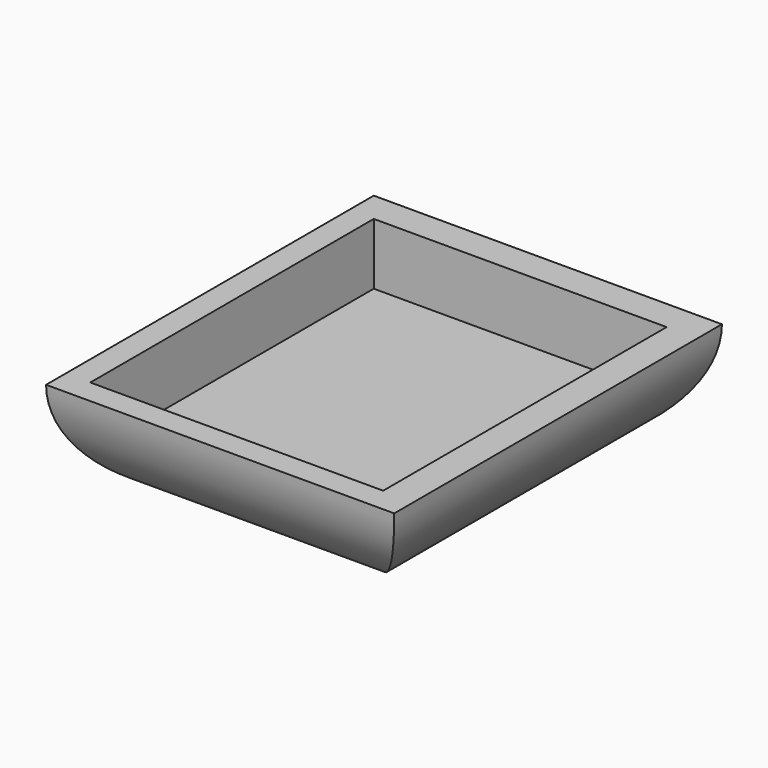
from build123d import *

# Parameters (mm, degrees)
F0_W     = 17
F0_H     = 20
F1_DEPTH = 5
F2_W     = 14.3
F2_H     = 17.3
F3_DEPTH = 3
F4_R     = 4.99999


# Not quite as in the source:
# - a fillet or chamfer is up to 0.001 mm smaller than in the source, because OpenCascade refuses the exact size


with BuildPart() as f1:
    # F0 (on Top) → F1 (new body)
    with BuildSketch(Plane.XY):
        with Locations((8.5, 10)):
            Rectangle(F0_W, F0_H)
    extrude(amount=F1_DEPTH)

    # F2 (on face) → F3 (cut)
    with BuildSketch(Plane.XY.offset(5)):
        with Locations((8.35, 9.85)):
            Rectangle(F2_W, F2_H)
    extrude(amount=-F3_DEPTH, mode=Mode.SUBTRACT)

    # F4 (radius 5 in the source; OpenCascade refuses exactly that, so slightly less here)
    f4_edges = [f1.edges().sort_by_distance(p)[0] for p in [
        (0, 10, 0),
        (8.5, 20, 0),
        (17, 10, 0),
        (8.5, 0, 0),
    ]]
    fillet(f4_edges, radius=F4_R)


solid = f1.part
